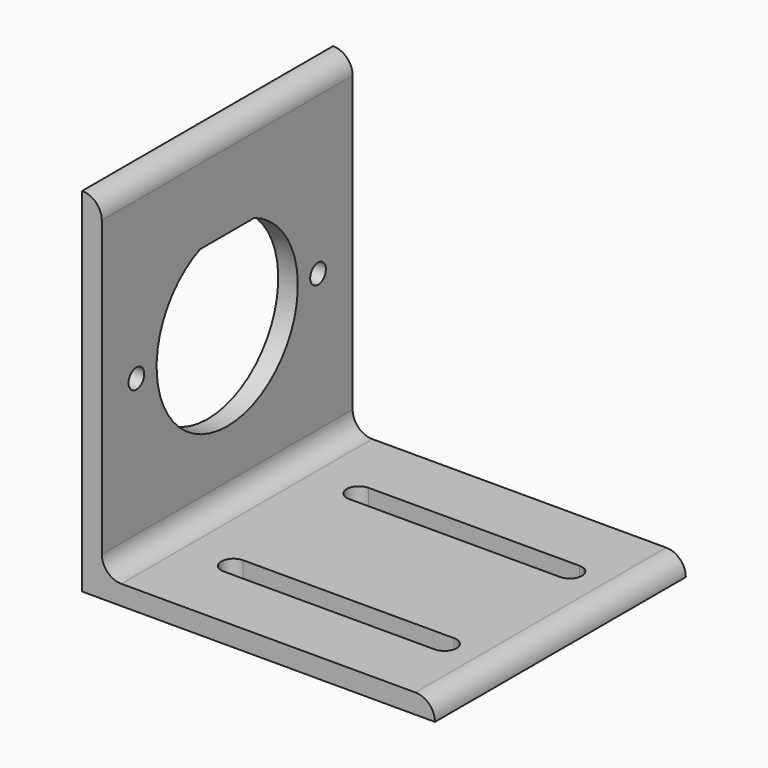
from build123d import *

# Parameters (mm, degrees)
F1_DEPTH = 101.6
F2_R     = 6.34999
F3_R     = 3.175
F4_DEPTH = 25.4
F6_DEPTH = 25.4


# Not quite as in the source:
# - a fillet or chamfer is up to 0.001 mm smaller than in the source, because OpenCascade refuses the exact size


with BuildPart() as f1:
    # F0 (on Front) → F1 (new body)
    with BuildSketch(Plane.XZ):
        Polygon((-79.5245949868, 52.4404040542), (-85.8745949868, 52.4404040542), (-85.8745949868, -61.8595959458), (28.4254050132, -61.8595959458), (28.4254050132, -55.5095959458), (-79.5245949868, -55.5095959458), align=None)
    extrude(amount=F1_DEPTH)

    # F2 (radius 6.35 in the source; OpenCascade refuses exactly that, so slightly less here)
    f2_edges = [f1.edges().sort_by_distance(p)[0] for p in [
        (-79.524595, -50.8, 52.440404),
        (28.425405, -50.8, -55.509596),
        (-79.524595, -50.8, -55.509596),
    ]]
    fillet(f2_edges, radius=F2_R)

    # F3 (on face) → F4 (cut)
    with BuildSketch(Plane.YZ.offset(-79.5245949868)):
        with BuildLine():
            Line((-39.7764292627, 21.6810040542), (-61.8235707373, 21.6810040542))
            ThreePointArc((-61.8235707373, 21.6810040542), (-50.8, -33.3099959458), (-39.7764292627, 21.6810040542))
        make_face()
        with Locations((-87.5792, -4.7095959458)):
            Circle(F3_R)
        with Locations((-14.0208, -4.7095959458)):
            Circle(F3_R)
    extrude(amount=-F4_DEPTH, mode=Mode.SUBTRACT)

    # F5 (on face) → F6 (cut)
    with BuildSketch(Plane.XY.offset(-55.5095959458)):
        with BuildLine():
            ThreePointArc((-57.1725949868, -72.263), (-61.1095949868, -76.2), (-57.1725949868, -80.137))
            Line((-57.1725949868, -80.137), (11.1534050132, -80.137))
            ThreePointArc((11.1534050132, -80.137), (15.0904050132, -76.2), (11.1534050132, -72.263))
            Line((11.1534050132, -72.263), (-57.1725949868, -72.263))
        make_face()
        with BuildLine():
            ThreePointArc((-57.1725949868, -21.463), (-61.1095949868, -25.4), (-57.1725949868, -29.337))
            Line((-57.1725949868, -29.337), (11.1534050132, -29.337))
            ThreePointArc((11.1534050132, -29.337), (15.0904050132, -25.4), (11.1534050132, -21.463))
            Line((11.1534050132, -21.463), (-57.1725949868, -21.463))
        make_face()
    extrude(amount=-F6_DEPTH, mode=Mode.SUBTRACT)


solid = f1.part
